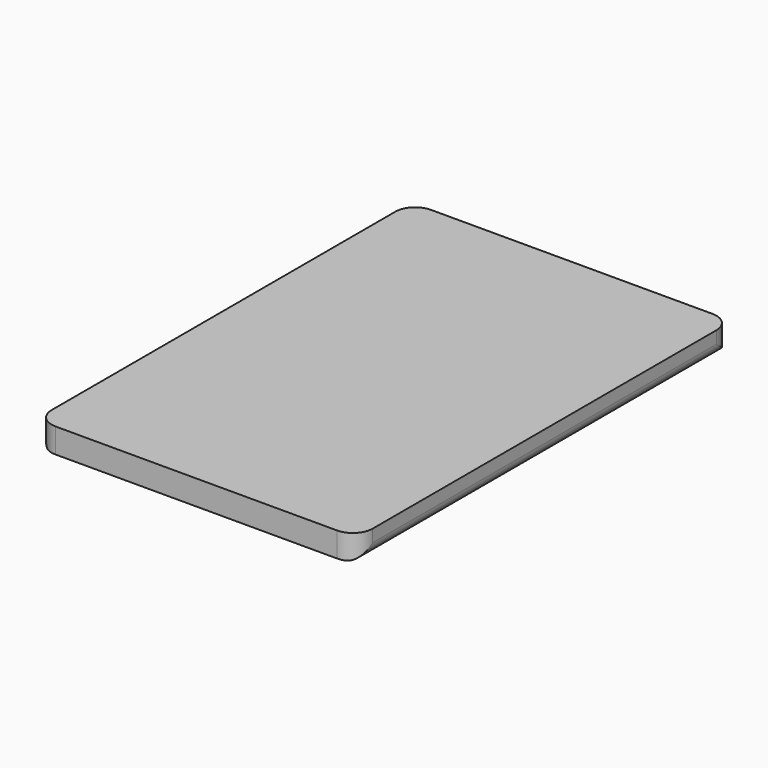
from build123d import *

# Parameters (mm, degrees)
F0_W        = 130
F0_H        = 190
F1_DEPTH    = 10
F2_T1_DEPTH = 49.9995000031
F3_T1_DEPTH = 199.0801997502


# Not quite as in the source:
# - a fillet or chamfer that OpenCascade refuses, or shapes differently, is made with other operations: its cross-section is extruded or revolved along the edge and cut away or added


with BuildPart() as f1:
    # F0 (on Top) → F1 (new body)
    with BuildSketch(Plane.XY):
        Rectangle(F0_W, F0_H)
    extrude(amount=F1_DEPTH)

    # F2: fillet of radius 8 on 4 edges, made by hand

    # F2_s2 → F2_t1 (cut)
    with BuildSketch(Plane.XY.offset(-19.9997500016)):
        with BuildLine():
            ThreePointArc((-65.0001, 87.0001), (-62.6569542495, 92.6569542495), (-57.0001, 95.0001))
            Line((-57.0001, 95.0001), (-57.0001, 95.1601))
            ThreePointArc((-57.0001, 95.1601), (-61.00005, 95.16), (-65, 95.16))
            Line((-65, 95.16), (-65.16, 95))
            ThreePointArc((-65.16, 95), (-65.16, 91.00005), (-65.1601, 87.0001))
            Line((-65.1601, 87.0001), (-65.0001, 87.0001))
        make_face()
        with BuildLine():
            ThreePointArc((65.0001, 87.0001), (62.6569542495, 92.6569542495), (57.0001, 95.0001))
            Line((57.0001, 95.0001), (57.0001, 95.1601))
            ThreePointArc((57.0001, 95.1601), (61.00005, 95.16), (65, 95.16))
            Line((65, 95.16), (65.16, 95))
            ThreePointArc((65.16, 95), (65.16, 91.00005), (65.1601, 87.0001))
            Line((65.1601, 87.0001), (65.0001, 87.0001))
        make_face()
        with BuildLine():
            ThreePointArc((57.0001, -95.0001), (62.6569542495, -92.6569542495), (65.0001, -87.0001))
            Line((65.0001, -87.0001), (65.1601, -87.0001))
            ThreePointArc((65.1601, -87.0001), (65.16, -91.00005), (65.16, -95))
            Line((65.16, -95), (65, -95.16))
            ThreePointArc((65, -95.16), (61.00005, -95.16), (57.0001, -95.1601))
            Line((57.0001, -95.1601), (57.0001, -95.0001))
        make_face()
        with BuildLine():
            ThreePointArc((-65.0001, -87.0001), (-62.6569542495, -92.6569542495), (-57.0001, -95.0001))
            Line((-57.0001, -95.0001), (-57.0001, -95.1601))
            ThreePointArc((-57.0001, -95.1601), (-61.00005, -95.16), (-65, -95.16))
            Line((-65, -95.16), (-65.16, -95))
            ThreePointArc((-65.16, -95), (-65.16, -91.00005), (-65.1601, -87.0001))
            Line((-65.1601, -87.0001), (-65.0001, -87.0001))
        make_face()
    extrude(amount=F2_T1_DEPTH, mode=Mode.SUBTRACT)

    # F3: fillet of radius 5 on 2 edges, made by hand

    # F3_s2 → F3_t1 (cut)
    with BuildSketch(Plane.XZ.offset(-99.5400998751)):
        with BuildLine():
            ThreePointArc((60, 0), (63.5355339059, 1.4644660941), (65, 5))
            Line((65, 5), (65, 0))
            Line((65, 0), (60, 0))
        make_face()
        with BuildLine():
            ThreePointArc((-65, 5), (-63.5355339059, 1.4644660941), (-60, 0))
            Line((-60, 0), (-65, 0))
            Line((-65, 0), (-65, 5))
        make_face()
    extrude(amount=F3_T1_DEPTH, mode=Mode.SUBTRACT)


solid = f1.part
